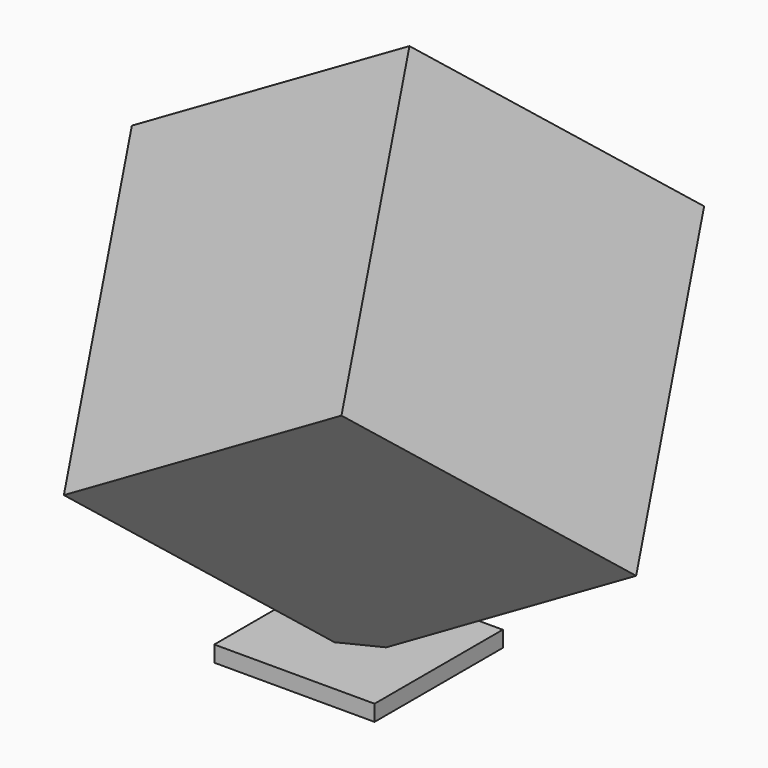
from build123d import *

# Parameters (mm, degrees)
F0_W     = 25
F0_H     = 25
F1_DEPTH = 2.5
F5_DEPTH = 50


# Not quite as in the source:
# - a feature of the source that left no trace in its solid (it failed there, or was rolled back) is left out


with BuildPart() as f1:
    # F0 (on Top) → F1 (new body)
    with BuildSketch(Plane.XY):
        Rectangle(F0_W, F0_H)
    extrude(amount=F1_DEPTH)

    # F4 (on line) → F5 (join)
    with BuildSketch(Plane(origin=(0, 0, 0), x_dir=(0, -1, 0), z_dir=(-0.8660254038, 0, -0.5))):
        Polygon((-35.3553390593, 35.3553390593), (0, 0), (35.3553390593, 35.3553390593), (0, 70.7106781187), align=None)
    extrude(amount=-F5_DEPTH)


solid = f1.part
